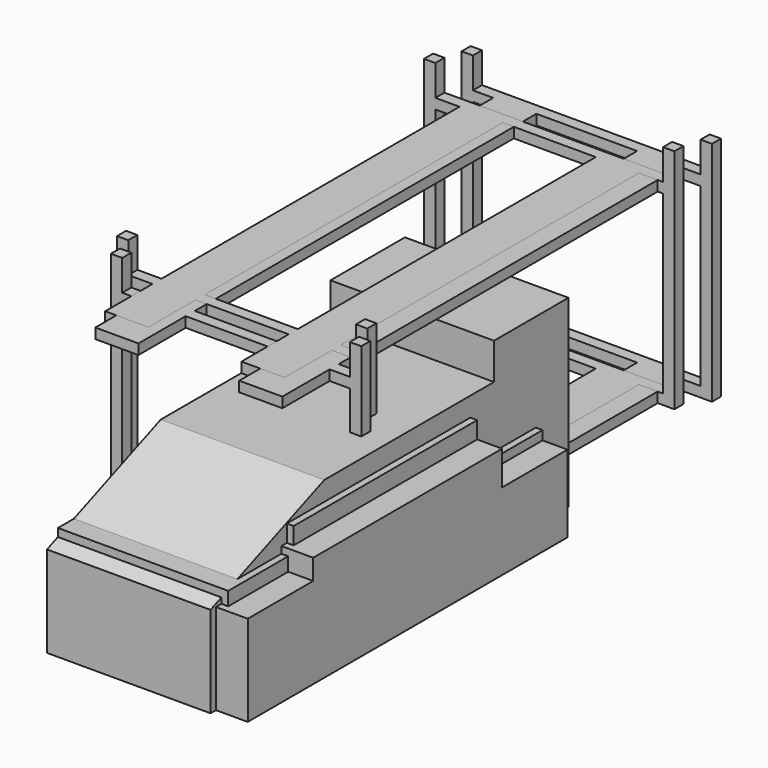
from build123d import *

# Parameters (mm, degrees)
F1_DEPTH  = 1905
F3_DEPTH  = 2184.4
F5_DEPTH  = 482.6
F6_W      = 596.9
F6_H      = 165.1
F7_DEPTH  = 254
F8_W      = 228.6
F8_H      = 355.6
F9_DEPTH  = 177.8
F10_W     = 215.9
F10_H     = 241.3
F11_DEPTH = 215.9
F13_DEPTH = 304.8
F14_W     = 203.2
F14_H     = 139.7
F15_DEPTH = 203.2
F16_W     = 749.3
F16_H     = 139.7
F17_DEPTH = 177.8
F18_W     = 336.55
F18_H     = 114.3
F19_DEPTH = 254
F20_W     = 285.75
F20_H     = 209.55
F21_DEPTH = 222.25
F22_W     = 298.45
F22_H     = 139.7
F23_DEPTH = 190.5
F24_W     = 412.75
F24_H     = 165.1
F25_DEPTH = 241.3
F26_W     = 139.7
F26_H     = 336.55
F27_DEPTH = 82.55
F28_W     = 304.8
F28_H     = 260.35
F29_DEPTH = 266.7
F30_W     = 438.15
F30_H     = 514.35
F31_DEPTH = 158.75
F32_W     = 203.2
F32_H     = 323.85
F33_DEPTH = 107.95
F34_W     = 114.3
F34_H     = 228.6
F35_DEPTH = 57.15
F36_W     = 292.1
F36_H     = 330.2
F37_DEPTH = 292.1
F39_DEPTH = 1828.8
F41_START = 2082.8
F40_W     = 227.0125
F40_H     = 127
F40_W_2   = 482.6
F40_W_3   = 1127.125
F40_H_2   = 4775.2
F40_H_3   = 660.4
F41_DEPTH = 114.3
F40_W_4   = 127
F42_DEPTH = 2540
F43_DEPTH = 114.3
F45_START = 2082.8
F44_W     = 269.875
F44_H     = 127
F44_W_2   = 482.6
F44_H_2   = 660.4
F44_H_3   = 4165.6
F44_W_3   = 1041.4
F45_DEPTH = 114.3
F44_W_4   = 127
F46_DEPTH = 2540
F47_DEPTH = 114.3


with BuildPart() as f1:
    # F0 (on Right) → F1 (new body)
    with BuildSketch(Plane.YZ):
        Polygon((-4394.2, 0), (0, 0), (0, 965.2), (-914.4, 965.2), (-914.4, 1435.1), (-3479.8, 1435.1), (-3479.8, 1168.4), (-4394.2, 1168.4), align=None)
    extrude(amount=F1_DEPTH)


with BuildPart() as f3:
    # F2 (on Right) → F3 (new body)
    with BuildSketch(Plane.YZ):
        Polygon((-4470.4, 0), (0, 0), (0, 863.6), (-914.4, 863.6), (-914.4, 1244.6), (-3556, 1244.6), (-3556, 1016), (-4470.4, 1016), align=None)
    extrude(amount=F3_DEPTH)


with BuildPart() as f5:
    # F4 (on Right) → F5 (new body)
    with BuildSketch(Plane.YZ):
        Polygon((-990.6, 0), (0, 0), (0, 177.8), (-914.4, 177.8), (-914.4, 1016), (-990.6, 1016), (-990.6, 177.8), align=None)
    extrude(amount=F5_DEPTH)


with BuildPart() as f7:
    # F6 (on Right) → F7 (new body)
    with BuildSketch(Plane.YZ):
        with Locations((-298.45, 82.55)):
            Rectangle(F6_W, F6_H)
    extrude(amount=F7_DEPTH)


with BuildPart() as f9:
    # F8 (on Right) → F9 (new body)
    with BuildSketch(Plane.YZ):
        with Locations((-114.3, 177.8)):
            Rectangle(F8_W, F8_H)
    extrude(amount=F9_DEPTH)


with BuildPart() as f11:
    # F10 (on Right) → F11 (new body)
    with BuildSketch(Plane.YZ):
        with Locations((-107.95, 120.65)):
            Rectangle(F10_W, F10_H)
    extrude(amount=F11_DEPTH)


with BuildPart() as f13:
    # F12 (on Right) → F13 (new body)
    with BuildSketch(Plane.YZ):
        Polygon((-76.2, 0), (0, 0), (0, 762), (-76.2, 254), align=None)
    extrude(amount=F13_DEPTH)


with BuildPart() as f15:
    # F14 (on Right) → F15 (new body)
    with BuildSketch(Plane.YZ):
        with Locations((-101.6, 64.134813758)):
            Rectangle(F14_W, F14_H)
    extrude(amount=F15_DEPTH)


with BuildPart() as f17:
    # F16 (on Right) → F17 (new body)
    with BuildSketch(Plane.YZ):
        with Locations((-374.65, 69.85)):
            Rectangle(F16_W, F16_H)
    extrude(amount=F17_DEPTH)


with BuildPart() as f19:
    # F18 (on Right) → F19 (new body)
    with BuildSketch(Plane.YZ):
        with Locations((-168.275, 57.15)):
            Rectangle(F18_W, F18_H)
    extrude(amount=F19_DEPTH)


with BuildPart() as f21:
    # F20 (on Right) → F21 (new body)
    with BuildSketch(Plane.YZ):
        with Locations((-142.875, 104.775)):
            Rectangle(F20_W, F20_H)
    extrude(amount=F21_DEPTH)


with BuildPart() as f23:
    # F22 (on Right) → F23 (new body)
    with BuildSketch(Plane.YZ):
        with Locations((-149.225, 69.85)):
            Rectangle(F22_W, F22_H)
    extrude(amount=F23_DEPTH)


with BuildPart() as f25:
    # F24 (on Right) → F25 (new body)
    with BuildSketch(Plane.YZ):
        with Locations((-206.375, 82.55)):
            Rectangle(F24_W, F24_H)
    extrude(amount=F25_DEPTH)


with BuildPart() as f27:
    # F26 (on Right) → F27 (new body)
    with BuildSketch(Plane.YZ):
        with Locations((-69.85, 168.275)):
            Rectangle(F26_W, F26_H)
    extrude(amount=F27_DEPTH)


with BuildPart() as f29:
    # F28 (on Right) → F29 (new body)
    with BuildSketch(Plane.YZ):
        with Locations((-152.4, 130.175)):
            Rectangle(F28_W, F28_H)
    extrude(amount=F29_DEPTH)


with BuildPart() as f31:
    # F30 (on Right) → F31 (new body)
    with BuildSketch(Plane.YZ):
        with Locations((-219.075, 257.175)):
            Rectangle(F30_W, F30_H)
    extrude(amount=F31_DEPTH)


with BuildPart() as f33:
    # F32 (on Right) → F33 (new body)
    with BuildSketch(Plane.YZ):
        with Locations((-101.6, 161.925)):
            Rectangle(F32_W, F32_H)
    extrude(amount=F33_DEPTH)


with BuildPart() as f35:
    # F34 (on Right) → F35 (new body)
    with BuildSketch(Plane.YZ):
        with Locations((-57.15, 114.3)):
            Rectangle(F34_W, F34_H)
    extrude(amount=F35_DEPTH)


with BuildPart() as f37:
    # F36 (on Right) → F37 (new body)
    with BuildSketch(Plane.YZ):
        with Locations((-146.05, 165.1)):
            Rectangle(F36_W, F36_H)
    extrude(amount=F37_DEPTH)


with BuildPart() as f39:
    # F38 (on Right) → F39 (new body)
    with BuildSketch(Plane.YZ):
        Polygon((-4546.6, 0), (0, 0), (0, 825.5), (-583.592414856, 1651), (-2956.2375545502, 1651), (-4546.6, 1018.8180208206), align=None)
        Polygon((0, 825.5), (0, 0), (457.2, 0), (457.2, 2057.4), (-583.592414856, 2057.4), (-583.592414856, 1651), align=None)
    extrude(amount=F39_DEPTH)


with BuildPart() as f41:
    # F40 (on Top) → F41 (new body)
    with BuildSketch(Plane.XY.offset(F41_START)):
        with Locations((1327.2400773999, -2049.0920517028)):
            Rectangle(F40_W, F40_H)
        with Locations((972.4338273999, -2049.0920517028)):
            Rectangle(F40_W_2, F40_H)
        with Locations((167.5713273999, -2049.0920517028)):
            Rectangle(F40_W_3, F40_H)
        with Locations((-637.2911726001, -2049.0920517028)):
            Rectangle(F40_W_2, F40_H)
        with Locations((-992.0974226001, -2049.0920517028)):
            Rectangle(F40_W, F40_H)
        with Locations((-637.2911726001, 402.0079482972)):
            Rectangle(F40_W_2, F40_H_2)
        with Locations((-637.2911726001, -2442.7920517028)):
            Rectangle(F40_W_2, F40_H_3)
        with Locations((972.4338273999, -2442.7920517028)):
            Rectangle(F40_W_2, F40_H_3)
        with Locations((972.4338273999, 402.0079482972)):
            Rectangle(F40_W_2, F40_H_2)
        with Locations((1327.2400773999, 2853.1079482972)):
            Rectangle(F40_W, F40_H)
        with Locations((972.4338273999, 2853.1079482972)):
            Rectangle(F40_W_2, F40_H)
        with Locations((167.5713273999, 2853.1079482972)):
            Rectangle(F40_W_3, F40_H)
        with Locations((-637.2911726001, 2853.1079482972)):
            Rectangle(F40_W_2, F40_H)
        with Locations((-992.0974226001, 2853.1079482972)):
            Rectangle(F40_W, F40_H)
    extrude(amount=F41_DEPTH)

    # F40 (on Top) → F42 (join)
    with BuildSketch(Plane.XY):
        with Locations((-1169.1036726001, -2049.0920517028)):
            Rectangle(F40_W_4, F40_H)
        with Locations((1504.2463273999, -2049.0920517028)):
            Rectangle(F40_W_4, F40_H)
        with Locations((1504.2463273999, 2853.1079482972)):
            Rectangle(F40_W_4, F40_H)
        with Locations((-1169.1036726001, 2853.1079482972)):
            Rectangle(F40_W_4, F40_H)
    extrude(amount=F42_DEPTH)

    # F40 (on Top) → F43 (join)
    with BuildSketch(Plane.XY):
        with Locations((-992.0974226001, -2049.0920517028)):
            Rectangle(F40_W, F40_H)
        with Locations((-637.2911726001, -2442.7920517028)):
            Rectangle(F40_W_2, F40_H_3)
        with Locations((-637.2911726001, -2049.0920517028)):
            Rectangle(F40_W_2, F40_H)
        with Locations((-637.2911726001, 402.0079482972)):
            Rectangle(F40_W_2, F40_H_2)
        with Locations((167.5713273999, -2049.0920517028)):
            Rectangle(F40_W_3, F40_H)
        with Locations((972.4338273999, -2442.7920517028)):
            Rectangle(F40_W_2, F40_H_3)
        with Locations((972.4338273999, -2049.0920517028)):
            Rectangle(F40_W_2, F40_H)
        with Locations((1327.2400773999, -2049.0920517028)):
            Rectangle(F40_W, F40_H)
        with Locations((972.4338273999, 402.0079482972)):
            Rectangle(F40_W_2, F40_H_2)
        with Locations((1327.2400773999, 2853.1079482972)):
            Rectangle(F40_W, F40_H)
        with Locations((972.4338273999, 2853.1079482972)):
            Rectangle(F40_W_2, F40_H)
        with Locations((167.5713273999, 2853.1079482972)):
            Rectangle(F40_W_3, F40_H)
        with Locations((-637.2911726001, 2853.1079482972)):
            Rectangle(F40_W_2, F40_H)
        with Locations((-992.0974226001, 2853.1079482972)):
            Rectangle(F40_W, F40_H)
    extrude(amount=F43_DEPTH)


with BuildPart() as f45:
    # F44 (on Top) → F45 (new body)
    with BuildSketch(Plane.XY.offset(F45_START)):
        with Locations((-1138.2375, -1754.857159253)):
            Rectangle(F44_W, F44_H)
        with Locations((-762, -1754.857159253)):
            Rectangle(F44_W_2, F44_H)
        with Locations((-762, -2148.557159253)):
            Rectangle(F44_W_2, F44_H_2)
        with Locations((-762, 391.442840747)):
            Rectangle(F44_W_2, F44_H_3)
        with Locations((0, -1754.857159253)):
            Rectangle(F44_W_3, F44_H)
        with Locations((762, -2148.557159253)):
            Rectangle(F44_W_2, F44_H_2)
        with Locations((762, -1754.857159253)):
            Rectangle(F44_W_2, F44_H)
        with Locations((1138.2375, -1754.857159253)):
            Rectangle(F44_W, F44_H)
        with Locations((762, 391.442840747)):
            Rectangle(F44_W_2, F44_H_3)
        with Locations((1138.2375, 2537.742840747)):
            Rectangle(F44_W, F44_H)
        with Locations((762, 2537.742840747)):
            Rectangle(F44_W_2, F44_H)
        with Locations((0, 2537.742840747)):
            Rectangle(F44_W_3, F44_H)
        with Locations((-762, 2537.742840747)):
            Rectangle(F44_W_2, F44_H)
        with Locations((-1138.2375, 2537.742840747)):
            Rectangle(F44_W, F44_H)
    extrude(amount=F45_DEPTH)

    # F44 (on Top) → F46 (join)
    with BuildSketch(Plane.XY):
        with Locations((-1336.675, -1754.857159253)):
            Rectangle(F44_W_4, F44_H)
        with Locations((1336.675, -1754.857159253)):
            Rectangle(F44_W_4, F44_H)
        with Locations((1336.675, 2537.742840747)):
            Rectangle(F44_W_4, F44_H)
        with Locations((-1336.675, 2537.742840747)):
            Rectangle(F44_W_4, F44_H)
    extrude(amount=F46_DEPTH)

    # F44 (on Top) → F47 (join)
    with BuildSketch(Plane.XY):
        with Locations((-762, 391.442840747)):
            Rectangle(F44_W_2, F44_H_3)
        with Locations((0, -1754.857159253)):
            Rectangle(F44_W_3, F44_H)
        with Locations((-762, 2537.742840747)):
            Rectangle(F44_W_2, F44_H)
        with Locations((762, -2148.557159253)):
            Rectangle(F44_W_2, F44_H_2)
        with Locations((-762, -2148.557159253)):
            Rectangle(F44_W_2, F44_H_2)
        with Locations((762, 2537.742840747)):
            Rectangle(F44_W_2, F44_H)
        with Locations((762, 391.442840747)):
            Rectangle(F44_W_2, F44_H_3)
        with Locations((0, 2537.742840747)):
            Rectangle(F44_W_3, F44_H)
        with Locations((762, -1754.857159253)):
            Rectangle(F44_W_2, F44_H)
        with Locations((-762, -1754.857159253)):
            Rectangle(F44_W_2, F44_H)
        with Locations((1138.2375, 2537.742840747)):
            Rectangle(F44_W, F44_H)
        with Locations((1138.2375, -1754.857159253)):
            Rectangle(F44_W, F44_H)
        with Locations((-1138.2375, 2537.742840747)):
            Rectangle(F44_W, F44_H)
        with Locations((-1138.2375, -1754.857159253)):
            Rectangle(F44_W, F44_H)
    extrude(amount=F47_DEPTH)


solid = Compound([f1.part, f3.part, f5.part, f7.part, f9.part, f11.part, f13.part, f15.part, f17.part, f19.part, f21.part, f23.part, f25.part, f27.part, f29.part, f31.part, f33.part, f35.part, f37.part, f39.part, f41.part, f45.part])
